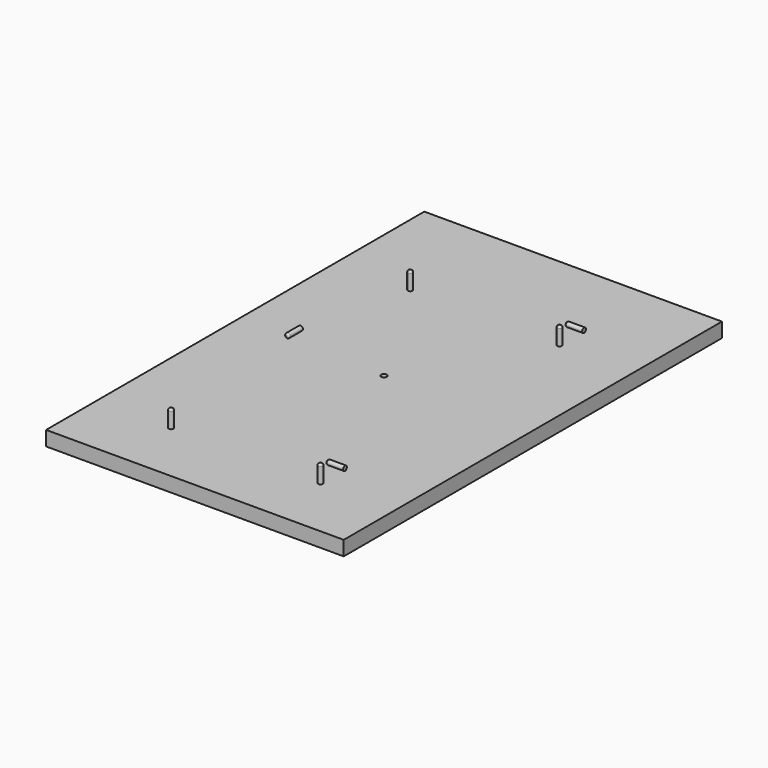
from build123d import *

# Parameters (mm, degrees)
F0_W      = 810
F0_H      = 25
F1_DEPTH  = 510
F3_D      = 10
F5_DEPTH  = 30
F6_R      = 3
F9_R      = 4
F10_DEPTH = 30
F11_R     = 3
F11_2_R   = 3
F13_DEPTH = 30


# Not quite as in the source:
# - a fillet or chamfer that OpenCascade refuses, or shapes differently, is made with other operations: its cross-section is extruded or revolved along the edge and cut away or added


with BuildPart() as f1:
    # F0 (on Right) → F1 (new body)
    with BuildSketch(Plane.YZ):
        with Locations((-405, 12.5)):
            Rectangle(F0_W, F0_H)
    extrude(amount=F1_DEPTH)

    # F3 (through all)
    with Locations(Plane.XY.offset(25)):
        with Locations((255, -405)):
            Hole(F3_D / 2)

    # F4 (on face) → F5 (join)
    with BuildSketch(Plane.XY.offset(25)):
        with BuildLine():
            ThreePointArc((131, -701), (129.8284271247, -698.1715728753), (127, -697))
            ThreePointArc((127, -697), (124.1715728753, -703.8284271247), (131, -701))
        make_face()
        with BuildLine():
            ThreePointArc((387, -701), (385.8284271247, -698.1715728753), (383, -697))
            ThreePointArc((383, -697), (380.1715728753, -703.8284271247), (387, -701))
        make_face()
        with BuildLine():
            ThreePointArc((387, -189), (380.1715728753, -186.1715728753), (383, -193))
            ThreePointArc((383, -193), (385.8284271247, -191.8284271247), (387, -189))
        make_face()
        with BuildLine():
            ThreePointArc((131, -189), (124.1715728753, -186.1715728753), (127, -193))
            ThreePointArc((127, -193), (129.8284271247, -191.8284271247), (131, -189))
        make_face()
    extrude(amount=F5_DEPTH)

    # F6
    f6_edges = [f1.edges().sort_by_distance(p)[0] for p in [
        (127, -705, 55),
        (383, -705, 55),
        (383, -185, 55),
        (127, -185, 55),
    ]]
    fillet(f6_edges, radius=F6_R)


with BuildPart() as f10:
    # F9 (on offset) → F10 (new body)
    with BuildSketch(Plane.YZ.offset(395)):
        with Locations((-701, 61)):
            Circle(F9_R)
    extrude(amount=F10_DEPTH)

    # F11
    f11_edges = [f10.edges().sort_by_distance(p)[0] for p in [
        (395, -705, 61),
    ]]
    fillet(f11_edges, radius=F11_R)


with BuildPart() as f10b:
    # F9 (on offset) → F10, piece 2 (new body)
    with BuildSketch(Plane.YZ.offset(395)):
        with BuildLine():
            Line((-189, 61), (-185, 61))
            ThreePointArc((-185, 61), (-189, 65), (-193, 61))
            Line((-193, 61), (-189, 61))
        make_face()
        with BuildLine():
            ThreePointArc((-193, 61), (-189, 57), (-185, 61))
            Line((-185, 61), (-189, 61))
            Line((-189, 61), (-193, 61))
        make_face()
    extrude(amount=F10_DEPTH)

    # F11#2
    f11_2_edges = [f10b.edges().sort_by_distance(p)[0] for p in [
        (395, -185, 61),
    ]]
    fillet(f11_2_edges, radius=F11_2_R)


with BuildPart() as f13:
    # F12 (on offset) → F13 (new body)
    with BuildSketch(Plane.XZ.offset(451.238)):
        with BuildLine():
            ThreePointArc((121, 61), (125, 57), (129, 61))
            ThreePointArc((129, 61), (125, 65), (121, 61))
        make_face()
    extrude(amount=-F13_DEPTH)

    # F14: fillet of radius 3 on 1 edges, made by hand

    # F14_s1 → F14_t2 (revolve, cut)
    with BuildSketch(Plane.XY.offset(61)):
        with BuildLine():
            ThreePointArc((121, -448.238), (121.8786796564, -450.3593203436), (124, -451.238))
            Line((124, -451.238), (121, -451.238))
            Line((121, -451.238), (121, -448.238))
        make_face()
    revolve(axis=Axis((125, -451.238, 61), (0, 1, 0)), mode=Mode.SUBTRACT)


solid = Compound([f1.part, f10.part, f10b.part, f13.part])
